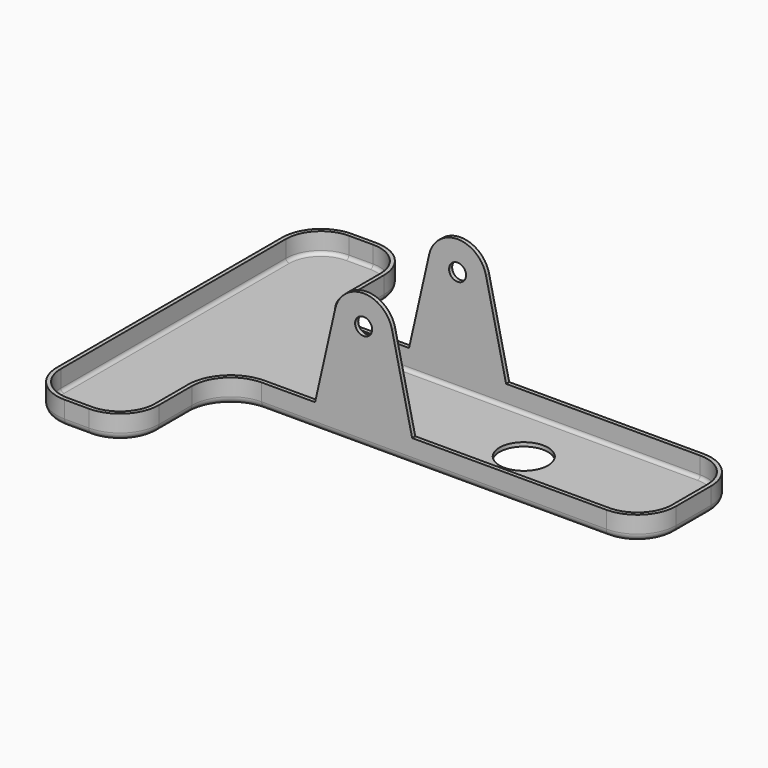
from build123d import *

# Parameters (mm, degrees)
F0_W      = 21
F0_H      = 24.5
F0_H_2    = 25
F0_R      = 5
F1_DEPTH  = 5
F2_R      = 8
F3_R      = 1.5
F4_T      = -0.8
F5_DEPTH  = 1.5
F7_DEPTH  = 0.8
F9_DEPTH  = 0.8
F11_DEPTH = 5
F12_R     = 0.99999


# Not quite as in the source:
# - a fillet or chamfer is up to 0.001 mm smaller than in the source, because OpenCascade refuses the exact size


with BuildPart() as f1:
    # F0 (on Top) → F1 (new body)
    with BuildSketch(Plane.XY):
        with Locations((-43.5, -24.75)):
            Rectangle(F0_W, F0_H)
        with Locations((-43.5, 0)):
            Rectangle(F0_W, F0_H_2)
        with Locations((-43.5, 24.75)):
            Rectangle(F0_W, F0_H)
        Polygon((54, 0), (54, 12.5), (-33, 12.5), (-33, -12.5), (54, -12.5), align=None)
        with Locations((19, 0)):
            Circle(F0_R, mode=Mode.SUBTRACT)
        with Locations((19, 0)):
            Circle(F0_R)
    extrude(amount=F1_DEPTH)

    # F2
    f2_edges = [f1.edges().sort_by_distance(p)[0] for p in [
        (-54, -37, 2.5),
        (-33, -37, 2.5),
        (-33, -12.5, 2.5),
        (54, 12.5, 2.5),
        (54, -12.5, 2.5),
        (-33, 37, 2.5),
        (-54, 37, 2.5),
        (-33, 12.5, 2.5),
    ]]
    fillet(f2_edges, radius=F2_R)

    # F3
    f3_edges = [f1.edges().sort_by_distance(p)[0] for p in [
        (-33, -24.75, 0),
        (-35.343146, -34.656854, 0),
        (-30.656854, -14.843146, 0),
        (-43.5, -37, 0),
        (10.5, -12.5, 0),
        (-51.656854, -34.656854, 0),
        (51.656854, -10.156854, 0),
        (-54, 0, 0),
        (54, 0, 0),
        (-51.656854, 34.656854, 0),
        (51.656854, 10.156854, 0),
        (-43.5, 37, 0),
        (10.5, 12.5, 0),
        (-35.343146, 34.656854, 0),
        (-30.656854, 14.843146, 0),
        (-33, 24.75, 0),
    ]]
    fillet(f3_edges, radius=F3_R)

    # F4
    f4_openings = [f1.faces().sort_by_distance(p)[0] for p in [
        (-12.15639, 0, 5),
    ]]
    offset(amount=F4_T, openings=f4_openings)

    # F0 (on Top) → F5 (cut, symmetric)
    with BuildSketch(Plane.XY):
        with Locations((19, 0)):
            Circle(F0_R)
    extrude(amount=F5_DEPTH, both=True, mode=Mode.SUBTRACT)

    # F6 (on face) → F7 (join)
    with BuildSketch(Plane.XZ.offset(12.5)):
        with BuildLine():
            ThreePointArc((2, 22), (1.9628709881, 22.6664604857), (1.8519434737, 23.3246726316))
            ThreePointArc((1.8519434737, 23.3246726316), (-4, 28), (-9.8519434737, 23.3246726316))
            ThreePointArc((-9.8519434737, 23.3246726316), (-8.6876452399, 18.2548722178), (-4, 16))
            ThreePointArc((-4, 16), (0.2426406871, 17.7573593129), (2, 22))
        make_face()
        with BuildLine():
            ThreePointArc((-2.25, 22), (-2.7625631329, 20.7625631329), (-4, 20.25))
            ThreePointArc((-4, 20.25), (-5.2374368671, 23.2374368671), (-2.25, 22))
        make_face(mode=Mode.SUBTRACT)
        with BuildLine():
            Line((-14, 5), (-4, 5))
            Line((-4, 5), (-4, 16))
            ThreePointArc((-4, 16), (-8.6876452399, 18.2548722178), (-9.8519434737, 23.3246726316))
            Line((-9.8519434737, 23.3246726316), (-14, 5))
        make_face()
        with BuildLine():
            Line((-4, 5), (6, 5))
            Line((6, 5), (1.8519434737, 23.3246726316))
            ThreePointArc((1.8519434737, 23.3246726316), (1.9628709881, 22.6664604857), (2, 22))
            ThreePointArc((2, 22), (0.2426406871, 17.7573593129), (-4, 16))
            Line((-4, 16), (-4, 5))
        make_face()
    extrude(amount=-F7_DEPTH)

    # F8 (on face) → F9 (join)
    with BuildSketch(Plane(origin=(0, 12.5, 0), x_dir=(-1, 0, 0), z_dir=(0, 1, 0))):
        with BuildLine():
            ThreePointArc((-1.8519434737, 23.3246726316), (-0.6876452399, 18.2548722178), (4, 16))
            ThreePointArc((4, 16), (8.2426406871, 17.7573593129), (10, 22))
            ThreePointArc((10, 22), (9.9628709881, 22.6664604857), (9.8519434737, 23.3246726316))
            ThreePointArc((9.8519434737, 23.3246726316), (4, 28), (-1.8519434737, 23.3246726316))
        make_face()
        with BuildLine():
            ThreePointArc((5.75, 22), (5.2374368671, 20.7625631329), (4, 20.25))
            ThreePointArc((4, 20.25), (2.7625631329, 23.2374368671), (5.75, 22))
        make_face(mode=Mode.SUBTRACT)
        with BuildLine():
            Line((4, 16), (4, 5))
            Line((4, 5), (14, 5))
            Line((14, 5), (9.8519434737, 23.3246726316))
            ThreePointArc((9.8519434737, 23.3246726316), (9.9628709881, 22.6664604857), (10, 22))
            ThreePointArc((10, 22), (8.2426406871, 17.7573593129), (4, 16))
        make_face()
        with BuildLine():
            Line((-6, 5), (4, 5))
            Line((4, 5), (4, 16))
            ThreePointArc((4, 16), (-0.6876452399, 18.2548722178), (-1.8519434737, 23.3246726316))
            Line((-1.8519434737, 23.3246726316), (-6, 5))
        make_face()
    extrude(amount=-F9_DEPTH)

    # F10 (on Front) → F11 (join, symmetric)
    with BuildSketch(Plane.XZ):
        with BuildLine():
            ThreePointArc((37.5, 0), (38.5, -1), (39.5, 0))
            Line((39.5, 0), (38.5, 0))
            Line((38.5, 0), (37.5, 0))
        make_face()
        with BuildLine():
            ThreePointArc((45.5, 0), (46.5, -1), (47.5, 0))
            Line((47.5, 0), (46.5, 0))
            Line((46.5, 0), (45.5, 0))
        make_face()
    extrude(amount=F11_DEPTH, both=True)

    # F12 (radius 1 in the source; OpenCascade refuses exactly that, so slightly less here)
    f12_edges = [f1.edges().sort_by_distance(p)[0] for p in [
        (46.5, -5, -1),
        (38.5, -5, -1),
        (46.5, 5, -1),
        (38.5, 5, -1),
    ]]
    fillet(f12_edges, radius=F12_R)


solid = f1.part
